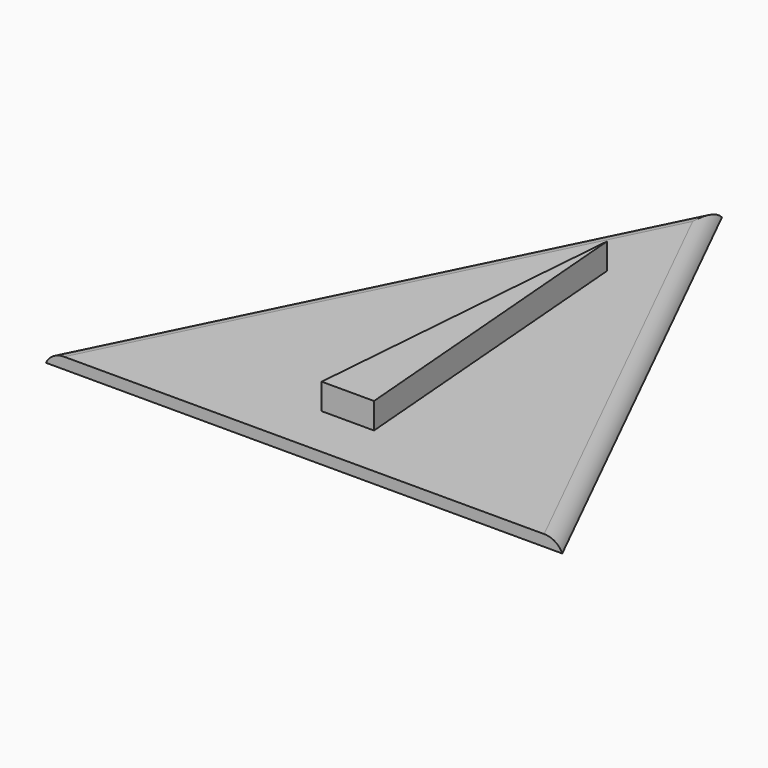
from build123d import *

# Parameters (mm, degrees)
F1_DEPTH    = 3.302
F2_T1_DEPTH = 194.5409515442
F2_T3_DEPTH = 194.4495264649
F4_DEPTH    = 7.62


# Not quite as in the source:
# - a fillet or chamfer that OpenCascade refuses, or shapes differently, is made with other operations: its cross-section is extruded or revolved along the edge and cut away or added


with BuildPart() as f1:
    # F0 (on Top) → F1 (new body)
    with BuildSketch(Plane.XY):
        Polygon((75.576454401, -75.9910270572), (0, 77.0177915692), (-75.7826715708, -75.9910270572), align=None)
    extrude(amount=F1_DEPTH)

    # F2: fillet of radius 5.08 on 2 edges, made by hand

    # F2_s2 → F2_t1 (cut)
    with BuildSketch(Plane(origin=(35.9116375184, 72.5073043447, 0), x_dir=(0, 0, 1), z_dir=(-0.4438288555, -0.8961115706, 0))):
        with BuildLine():
            ThreePointArc((0, 34.1827182836), (2.3956458882, 32.3200753886), (3.302, 29.4240298088))
            Line((3.302, 29.4240298088), (3.302, 34.1827182836))
            Line((3.302, 34.1827182836), (0, 34.1827182836))
        make_face()
    extrude(amount=F2_T1_DEPTH, mode=Mode.SUBTRACT)

    # F2_s4 → F2_t3 (cut)
    with BuildSketch(Plane(origin=(50.2640998489, -101.7625211206, 0), x_dir=(0, 0, 1), z_dir=(-0.4428582479, 0.8965916418, 0))):
        with BuildLine():
            ThreePointArc((0, 34.1079642346), (2.3956458882, 32.2453213396), (3.302, 29.3492757599))
            Line((3.302, 29.3492757599), (3.302, 34.1079642346))
            Line((3.302, 34.1079642346), (0, 34.1079642346))
        make_face()
    extrude(amount=F2_T3_DEPTH, mode=Mode.SUBTRACT)

    # F3 (on face) → F4 (join)
    with BuildSketch(Plane.XY.offset(3.302)):
        Polygon((7.7744186856, -60.2337494493), (0, 34.9251665175), (-7.5671025552, -60.2337494493), align=None)
    extrude(amount=F4_DEPTH)


solid = f1.part
